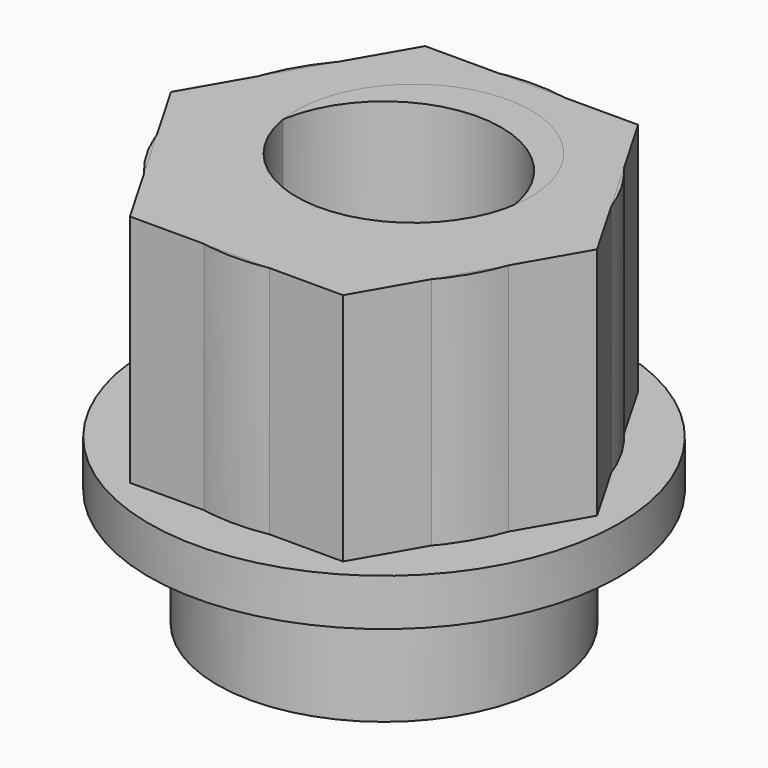
from build123d import *

# Parameters (mm, degrees)
F0_R     = 4
F0_R_2   = 2.5
F1_DEPTH = 1
F2_DEPTH = 6
F3_R     = 3.555
F3_R_2   = 2.5
F4_DEPTH = 6
F5_DEPTH = 1
F6_DEPTH = 2.5


with BuildPart() as f1:
    # F0 (on Top) → F1 (new body)
    with BuildSketch(Plane.XY):
        Circle(F0_R)
        Circle(F0_R_2, mode=Mode.SUBTRACT)
    extrude(amount=F1_DEPTH)


with BuildPart() as f2:
    # F0 (on Top) → F2 (new body)
    with BuildSketch(Plane.XY):
        Circle(F0_R)
        Circle(F0_R_2, mode=Mode.SUBTRACT)
    extrude(amount=F2_DEPTH)


with BuildPart() as f4:
    # F3 (on Top) → F4 (new body)
    with BuildSketch(Plane.XY):
        Polygon((-2.2718733093, -3.935), (2.2718733093, -3.935), (4.5437466185, 0), (2.2718733093, 3.935), (-2.2718733093, 3.935), (-4.5437466185, 0), align=None)
        Circle(F3_R, mode=Mode.SUBTRACT)
        Circle(F3_R)
        with Locations((0, 0.79)):
            Circle(F3_R_2, mode=Mode.SUBTRACT)
    extrude(amount=F4_DEPTH)

    # F3 (on Top) → F5 (join)
    with BuildSketch(Plane.XY):
        with BuildLine():
            Line((0, 4.2109526637), (-1.705, 4.7109526637))
            ThreePointArc((-1.705, 4.7109526637), (0, -5.01), (1.705, 4.7109526637))
            Line((1.705, 4.7109526637), (0, 4.2109526637))
        make_face()
        Polygon((4.5437466185, 0), (2.2718733093, -3.935), (-2.2718733093, -3.935), (-4.5437466185, 0), (-2.2718733093, 3.935), (2.2718733093, 3.935), align=None, mode=Mode.SUBTRACT)
    extrude(amount=F5_DEPTH)

    # F3 (on Top) → F6 (join)
    with BuildSketch(Plane.XY):
        Circle(F3_R)
        with Locations((0, 0.79)):
            Circle(F3_R_2, mode=Mode.SUBTRACT)
    extrude(amount=-F6_DEPTH)


solid = Compound([f1.part, f2.part, f4.part])
